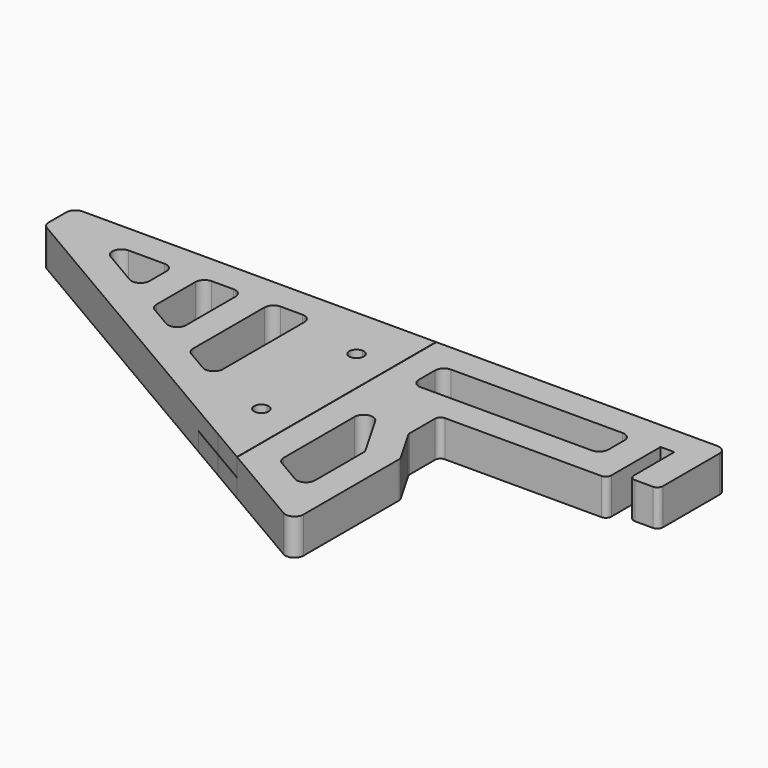
from build123d import *

# Parameters (mm, degrees)
F0_W     = 104.4
F0_H     = 21
F1_DEPTH = 20
F2_DEPTH = 9.9
F3_DEPTH = 20
F4_DEPTH = 10.1
F5_DEPTH = 0.2
F6_R     = 5
F6_2_R   = 5
F7_R     = 3


with BuildPart() as f1:
    # F0 (on Top) → F1 (new body)
    with BuildSketch(Plane.XY):
        Polygon((155.8509568507, -10.3563018057), (155.8509568507, 36.6436981943), (-4.1490431493, 36.6436981943), (-4.1490431493, -100.6021034165), (51.5509568507, -133.2550591652), (51.5509568507, -57.7480911735), (39.9509568507, -37.6563018057), (39.9509568507, -16.3563018057), (132.2509568507, -16.3563018057), (132.2509568507, 20.6436981943), (139.8509568507, 20.6436981943), (139.8509568507, -10.3563018057), align=None)
        Polygon((11.8509568507, -91.4351209706), (11.8509568507, -20.985674113), (35.5509568507, -62.0352782524), (35.5509568507, -105.3287484615), align=None, mode=Mode.SUBTRACT)
        with Locations((64.0509568507, 10.1436981943)):
            Rectangle(F0_W, F0_H, mode=Mode.SUBTRACT)
    extrude(amount=F1_DEPTH)

    # F0 (on Top) → F2 (join)
    with BuildSketch(Plane.XY):
        with BuildLine():
            Line((-4.1490431493, -100.6021034165), (-4.1490431493, 36.6436981943))
            Line((-4.1490431493, 36.6436981943), (-24.1490431493, 36.6436981943))
            Line((-24.1490431493, 36.6436981943), (-24.1490431493, 10.6436981943))
            ThreePointArc((-24.1490431493, 10.6436981943), (-21.3206160245, 9.472125319), (-20.1490431493, 6.6436981943))
            ThreePointArc((-20.1490431493, 6.6436981943), (-21.3206160245, 3.8152710695), (-24.1490431493, 2.6436981943))
            Line((-24.1490431493, 2.6436981943), (-24.1490431493, -54.8775232555))
            ThreePointArc((-24.1490431493, -54.8775232555), (-21.3206160245, -56.0490961307), (-20.1490431493, -58.8775232555))
            ThreePointArc((-20.1490431493, -58.8775232555), (-21.3206160245, -61.7059503802), (-24.1490431493, -62.8775232555))
            Line((-24.1490431493, -62.8775232555), (-24.1490431493, -88.8775232555))
            Line((-24.1490431493, -88.8775232555), (-4.1490431493, -100.6021034165))
        make_face()
        with BuildLine():
            Line((-24.1490431493, 10.6436981943), (-24.1490431493, 36.6436981943))
            Line((-24.1490431493, 36.6436981943), (-44.1490431493, 36.6436981943))
            Line((-44.1490431493, 36.6436981943), (-44.1490431493, -77.1529430944))
            Line((-44.1490431493, -77.1529430944), (-24.1490431493, -88.8775232555))
            Line((-24.1490431493, -88.8775232555), (-24.1490431493, -62.8775232555))
            ThreePointArc((-24.1490431493, -62.8775232555), (-28.1490431493, -58.8775232555), (-24.1490431493, -54.8775232555))
            Line((-24.1490431493, -54.8775232555), (-24.1490431493, 2.6436981943))
            ThreePointArc((-24.1490431493, 2.6436981943), (-28.1490431493, 6.6436981943), (-24.1490431493, 10.6436981943))
        make_face()
    extrude(amount=F2_DEPTH)

    # F6
    f6_edges = [f1.edges().sort_by_distance(p)[0] for p in [
        (35.550957, -105.328748, 10),
        (11.850957, -91.435121, 10),
        (11.850957, -20.985674, 10),
        (35.550957, -62.035278, 10),
        (11.850957, 20.643698, 10),
        (11.850957, -0.356302, 10),
        (116.250957, -0.356302, 10),
        (116.250957, 20.643698, 10),
        (155.850957, 36.643698, 10),
        (51.550957, -133.255059, 10),
    ]]
    fillet(f6_edges, radius=F6_R)

    # F7
    f7_edges = [f1.edges().sort_by_distance(p)[0] for p in [
        (132.250957, -16.356302, 10),
        (139.850957, -10.356302, 10),
        (155.850957, -10.356302, 10),
        (51.550957, -57.748091, 10),
        (39.950957, -37.656302, 10),
        (39.950957, -16.356302, 10),
    ]]
    fillet(f7_edges, radius=F7_R)


with BuildPart() as f3:
    # F0 (on Top) → F3 (new body)
    with BuildSketch(Plane.XY):
        Polygon((-44.1490431493, -77.1529430944), (-44.1490431493, 36.6436981943), (-204.1490431493, 36.6436981943), (-204.1490431493, 16.6436981943), align=None)
        Polygon((-82.1490431493, 20.6436981943), (-60.1490431493, 20.6436981943), (-60.1490431493, -49.2266323907), (-82.1490431493, -36.3295942135), (-98.1490431493, -26.9499300847), (-120.1490431493, -14.0528919075), (-136.1490431493, -4.6732277786), (-179.335111435, 20.6436981943), (-136.1490431493, 20.6436981943), (-120.1490431493, 20.6436981943), (-98.1490431493, 20.6436981943), align=None, mode=Mode.SUBTRACT)
        with BuildLine():
            Line((-4.1490431493, -100.6021034165), (-4.1490431493, 36.6436981943))
            Line((-4.1490431493, 36.6436981943), (-24.1490431493, 36.6436981943))
            Line((-24.1490431493, 36.6436981943), (-24.1490431493, 10.6436981943))
            ThreePointArc((-24.1490431493, 10.6436981943), (-21.3206160245, 9.472125319), (-20.1490431493, 6.6436981943))
            ThreePointArc((-20.1490431493, 6.6436981943), (-21.3206160245, 3.8152710695), (-24.1490431493, 2.6436981943))
            Line((-24.1490431493, 2.6436981943), (-24.1490431493, -54.8775232555))
            ThreePointArc((-24.1490431493, -54.8775232555), (-21.3206160245, -56.0490961307), (-20.1490431493, -58.8775232555))
            ThreePointArc((-20.1490431493, -58.8775232555), (-21.3206160245, -61.7059503802), (-24.1490431493, -62.8775232555))
            Line((-24.1490431493, -62.8775232555), (-24.1490431493, -88.8775232555))
            Line((-24.1490431493, -88.8775232555), (-4.1490431493, -100.6021034165))
        make_face()
        with BuildLine():
            Line((-24.1490431493, 10.6436981943), (-24.1490431493, 36.6436981943))
            Line((-24.1490431493, 36.6436981943), (-44.1490431493, 36.6436981943))
            Line((-44.1490431493, 36.6436981943), (-44.1490431493, -77.1529430944))
            Line((-44.1490431493, -77.1529430944), (-24.1490431493, -88.8775232555))
            Line((-24.1490431493, -88.8775232555), (-24.1490431493, -62.8775232555))
            ThreePointArc((-24.1490431493, -62.8775232555), (-28.1490431493, -58.8775232555), (-24.1490431493, -54.8775232555))
            Line((-24.1490431493, -54.8775232555), (-24.1490431493, 2.6436981943))
            ThreePointArc((-24.1490431493, 2.6436981943), (-28.1490431493, 6.6436981943), (-24.1490431493, 10.6436981943))
        make_face()
        Polygon((-120.1490431493, -14.0528919075), (-120.1490431493, 20.6436981943), (-136.1490431493, 20.6436981943), (-136.1490431493, -4.6732277786), align=None)
        Polygon((-82.1490431493, -36.3295942135), (-82.1490431493, 20.6436981943), (-98.1490431493, 20.6436981943), (-98.1490431493, -26.9499300847), align=None)
    extrude(amount=F3_DEPTH)

    # F0 (on Top) → F4 (cut)
    with BuildSketch(Plane.XY):
        with BuildLine():
            Line((-24.1490431493, 10.6436981943), (-24.1490431493, 36.6436981943))
            Line((-24.1490431493, 36.6436981943), (-44.1490431493, 36.6436981943))
            Line((-44.1490431493, 36.6436981943), (-44.1490431493, -77.1529430944))
            Line((-44.1490431493, -77.1529430944), (-24.1490431493, -88.8775232555))
            Line((-24.1490431493, -88.8775232555), (-24.1490431493, -62.8775232555))
            ThreePointArc((-24.1490431493, -62.8775232555), (-28.1490431493, -58.8775232555), (-24.1490431493, -54.8775232555))
            Line((-24.1490431493, -54.8775232555), (-24.1490431493, 2.6436981943))
            ThreePointArc((-24.1490431493, 2.6436981943), (-28.1490431493, 6.6436981943), (-24.1490431493, 10.6436981943))
        make_face()
        with BuildLine():
            Line((-4.1490431493, -100.6021034165), (-4.1490431493, 36.6436981943))
            Line((-4.1490431493, 36.6436981943), (-24.1490431493, 36.6436981943))
            Line((-24.1490431493, 36.6436981943), (-24.1490431493, 10.6436981943))
            ThreePointArc((-24.1490431493, 10.6436981943), (-21.3206160245, 9.472125319), (-20.1490431493, 6.6436981943))
            ThreePointArc((-20.1490431493, 6.6436981943), (-21.3206160245, 3.8152710695), (-24.1490431493, 2.6436981943))
            Line((-24.1490431493, 2.6436981943), (-24.1490431493, -54.8775232555))
            ThreePointArc((-24.1490431493, -54.8775232555), (-21.3206160245, -56.0490961307), (-20.1490431493, -58.8775232555))
            ThreePointArc((-20.1490431493, -58.8775232555), (-21.3206160245, -61.7059503802), (-24.1490431493, -62.8775232555))
            Line((-24.1490431493, -62.8775232555), (-24.1490431493, -88.8775232555))
            Line((-24.1490431493, -88.8775232555), (-4.1490431493, -100.6021034165))
        make_face()
    extrude(amount=F4_DEPTH, mode=Mode.SUBTRACT)

    # F5 (cut): faces of the model
    f5_faces = [f3.faces().sort_by_distance(p)[0] for p in [
        (-44.1490431493, -20.2546224501, 5.05),
        (-4.1490431493, -31.9792026111, 15.05),
    ]]
    extrude(f5_faces, amount=-F5_DEPTH, mode=Mode.SUBTRACT)

    # F6#2
    f6_2_edges = [f3.edges().sort_by_distance(p)[0] for p in [
        (-179.335111, 20.643698, 10),
        (-136.149043, 20.643698, 10),
        (-136.149043, -4.673228, 10),
        (-98.149043, -26.94993, 10),
        (-98.149043, 20.643698, 10),
        (-120.149043, 20.643698, 10),
        (-120.149043, -14.052892, 10),
        (-60.149043, 20.643698, 10),
        (-60.149043, -49.226632, 10),
        (-82.149043, -36.329594, 10),
        (-82.149043, 20.643698, 10),
        (-204.149043, 16.643698, 10),
        (-204.149043, 36.643698, 10),
    ]]
    fillet(f6_2_edges, radius=F6_2_R)


solid = Compound([f1.part, f3.part])
